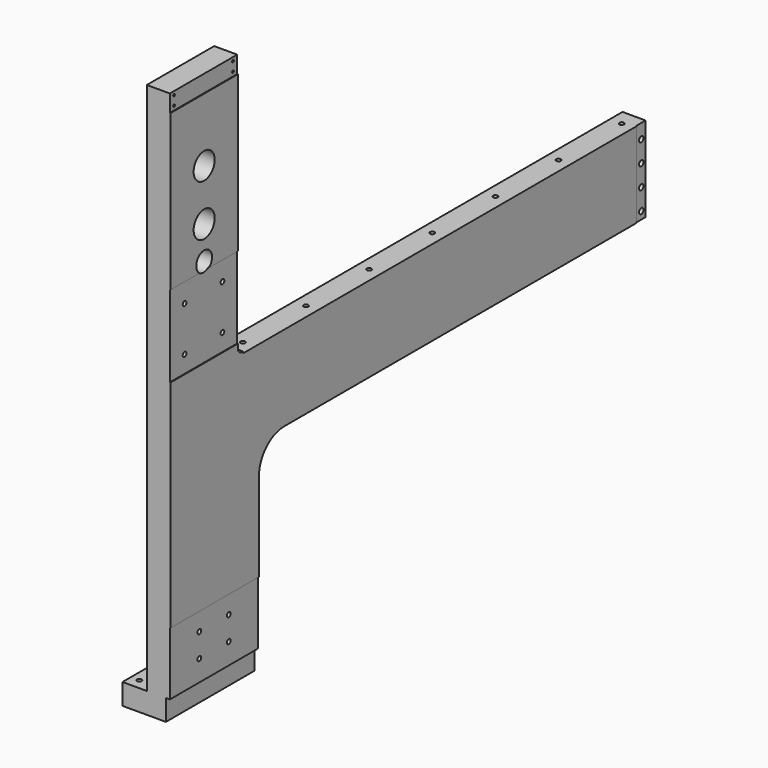
from build123d import *

# Parameters (mm, degrees)
F0_R      = 63.5
F1_DEPTH  = 57.15
F2_W      = 406.4
F2_H      = 82.55
F3_DEPTH  = 3.048
F5_D      = 10.71626
F5_DEPTH  = 25.4
F5_TIP    = 3.2194893086
F8_D      = 22.225
F8_DEPTH  = 50.8
F8_TIP    = 6.6770636289
F9_W      = 57.15
F9_H      = 411.099
F10_DEPTH = 3.175
F12_D     = 26.924
F14_D     = 22.225
F14_DEPTH = 50.8
F14_TIP   = 6.6770636289
F15_W     = 533.4
F15_H     = 304.8
F16_DEPTH = 3.048
F18_D     = 22.225
F18_DEPTH = 50.8
F18_TIP   = 6.6770636289
F20_W     = 533.4
F20_H     = 101.6
F21_DEPTH = 209.55
F23_D     = 22.225
F24_W     = 282.4820266962
F24_H     = 393.7
F24_W_2   = 406.4
F24_R     = 11.1125
F24_W_3   = 225.5179733038
F25_DEPTH = 3.048
F26_R     = 47.625
F27_DEPTH = 114.301
F28_W     = 190.5
F28_H     = 127
F28_R     = 47.625
F29_DEPTH = 12.7
F31_D     = 13.49248
F31_DEPTH = 31.75
F31_TIP   = 4.0535499425


with BuildPart() as f1:
    # F0 (on Right) → F1 (new body, symmetric)
    with BuildSketch(Plane.YZ):
        with BuildLine():
            Line((406.4, 1338.326), (0, 1338.326))
            Line((0, 1338.326), (0, 65.024))
            Line((0, 65.024), (0, -354.076))
            Line((0, -354.076), (0, -642.7685022354))
            Line((0, -642.7685022354), (0, -1236.726))
            Line((0, -1236.726), (533.4, -1236.726))
            Line((533.4, -1236.726), (533.4, -506.476))
            ThreePointArc((533.4, -506.476), (578.0369265472, -398.7129265472), (685.8, -354.076))
            Line((685.8, -354.076), (2870.2, -354.076))
            Line((2870.2, -354.076), (2870.2, 57.023))
            Line((2870.2, 57.023), (438.15, 57.023))
            Line((438.15, 57.023), (438.15, 65.024))
            Line((438.15, 65.024), (431.8, 65.024))
            ThreePointArc((431.8, 65.024), (413.8394877579, 72.4634877579), (406.4, 90.424))
            Line((406.4, 90.424), (406.4, 1338.326))
        make_face()
        with Locations((203.2, 701.548)):
            Circle(F0_R, mode=Mode.SUBTRACT)
        with Locations((203.2, 949.198)):
            Circle(F0_R, mode=Mode.SUBTRACT)
    extrude(amount=F1_DEPTH, both=True)

    # F2 (on face) → F3 (cut)
    with BuildSketch(Plane.YZ.offset(57.15)):
        with Locations((203.2, 1297.051)):
            Rectangle(F2_W, F2_H)
    extrude(amount=-F3_DEPTH, mode=Mode.SUBTRACT)

    # F5
    with Locations(Plane.YZ.offset(54.102)):
        with Locations((25.4, 1320.673), (25.4, 1276.223), (381, 1320.673), (381, 1276.223)):
            Hole(F5_D / 2, depth=F5_DEPTH)
            with Locations((0, 0, -(F5_DEPTH + F5_TIP / 2))):  # 118° drill point
                Cone(0, F5_D / 2, F5_TIP, mode=Mode.SUBTRACT)

    # F8
    with Locations(Plane.YZ.offset(57.15)):
        with Locations((88.9, 409.448), (317.5, 409.448), (88.9, 193.548), (317.5, 193.548)):
            Hole(F8_D / 2, depth=F8_DEPTH)
            with Locations((0, 0, -(F8_DEPTH + F8_TIP / 2))):  # 118° drill point
                Cone(0, F8_D / 2, F8_TIP, mode=Mode.SUBTRACT)

    # F9 (on face) → F10 (cut)
    with BuildSketch(Plane.YZ.offset(57.15)):
        with Locations((2841.625, -148.5265)):
            Rectangle(F9_W, F9_H)
    extrude(amount=-F10_DEPTH, mode=Mode.SUBTRACT)

    # F12 (through all)
    with Locations(Plane.YZ.offset(53.975)):
        with Locations((2844.8, -12.827), (2844.8, -114.427), (2844.8, -216.027), (2844.8, -317.627)):
            Hole(F12_D / 2)

    # F14
    with Locations(Plane.XY.offset(57.023)):
        with Locations((0, 508), (0, 889), (0, 1270), (0, 1651), (0, 2032), (0, 2413), (0, 2794)):
            Hole(F14_D / 2, depth=F14_DEPTH)
            with Locations((0, 0, -(F14_DEPTH + F14_TIP / 2))):  # 118° drill point
                Cone(0, F14_D / 2, F14_TIP, mode=Mode.SUBTRACT)

    # F15 (on face) → F16 (cut)
    with BuildSketch(Plane.YZ.offset(57.15)):
        with Locations((266.7, -1084.326)):
            Rectangle(F15_W, F15_H)
    extrude(amount=-F16_DEPTH, mode=Mode.SUBTRACT)

    # F18
    with Locations(Plane.YZ.offset(54.102)):
        with Locations((177.8, -1020.826), (355.6, -1020.826), (355.6, -1135.126), (177.8, -1135.126)):
            Hole(F18_D / 2, depth=F18_DEPTH)
            with Locations((0, 0, -(F18_DEPTH + F18_TIP / 2))):  # 118° drill point
                Cone(0, F18_D / 2, F18_TIP, mode=Mode.SUBTRACT)

    # F20 (on offset) → F21 (join)
    with BuildSketch(Plane.YZ.offset(35.052)):
        with Locations((266.7, -1287.526)):
            Rectangle(F20_W, F20_H)
    extrude(amount=-F21_DEPTH)

    # F23 (through all)
    with Locations(Plane(origin=(0, 0, -1338.326), x_dir=(1, 0, 0), z_dir=(0, 0, -1))):
        with Locations((-133.35, -482.6), (-133.35, -266.7), (-133.35, -50.8)):
            Hole(F23_D / 2)

    # F24 (on face) → F25 (cut)
    with BuildSketch(Plane.YZ.offset(57.15)):
        with Locations((547.6410133481, 307.848)):
            Rectangle(F24_W, F24_H)
        with Locations((203.2, 307.848)):
            Rectangle(F24_W_2, F24_H)
        with Locations((88.9, 193.548)):
            Circle(F24_R, mode=Mode.SUBTRACT)
        with Locations((88.9, 409.448)):
            Circle(F24_R, mode=Mode.SUBTRACT)
        with Locations((317.5, 193.548)):
            Circle(F24_R, mode=Mode.SUBTRACT)
        with Locations((317.5, 409.448)):
            Circle(F24_R, mode=Mode.SUBTRACT)
        with Locations((-112.7589866519, 307.848)):
            Rectangle(F24_W_3, F24_H)
    extrude(amount=-F25_DEPTH, mode=Mode.SUBTRACT)

    # F26 (on face) → F27 (cut, through all)
    with BuildSketch(Plane(origin=(-57.15, 0, 0), x_dir=(0, -1, 0), z_dir=(-1, 0, 0))):
        with Locations((-203.2, 542.798)):
            Circle(F26_R)
    extrude(amount=-F27_DEPTH, mode=Mode.SUBTRACT)

    # F28 (on face) → F29 (join)
    with BuildSketch(Plane(origin=(-57.15, 0, 0), x_dir=(0, -1, 0), z_dir=(-1, 0, 0))):
        with Locations((-203.2, 542.798)):
            Rectangle(F28_W, F28_H)
        with Locations((-203.2, 542.798)):
            Circle(F28_R, mode=Mode.SUBTRACT)
    extrude(amount=F29_DEPTH)

    # F31
    with Locations(Plane(origin=(-69.85, 0, 0), x_dir=(0, -1, 0), z_dir=(-1, 0, 0))):
        with Locations((-276.352, 585.724), (-130.048, 585.724), (-130.048, 499.872), (-276.352, 499.872)):
            Hole(F31_D / 2, depth=F31_DEPTH)
            with Locations((0, 0, -(F31_DEPTH + F31_TIP / 2))):  # 118° drill point
                Cone(0, F31_D / 2, F31_TIP, mode=Mode.SUBTRACT)


solid = f1.part
